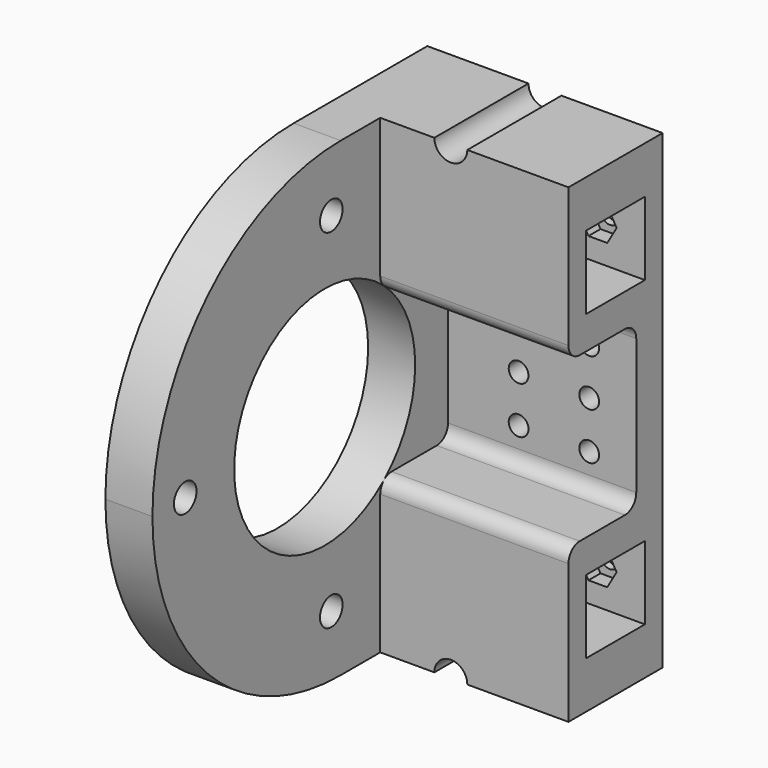
from build123d import *

# Parameters (mm, degrees)
F1_DEPTH     = 100
F2_W         = 15.6
F2_H         = 15.6
F3_DEPTH     = 134.9
F5_DEPTH     = 3.2
F6_R         = 2.025
F7_DEPTH     = 10
F8_R         = 3
F8_R_2       = 24.0417525773
F9_DEPTH     = 15
F10_R        = 49.99999
F11_W        = 18
F11_H        = 34.8
F12_DEPTH    = 100
F13_R        = 3.5
F14_DEPTH    = 50
F15_R        = 2.1
F16_DEPTH    = 25
F17_T1_DEPTH = 47.5
F17_T3_DEPTH = 47.5


# Not quite as in the source:
# - a fillet or chamfer that OpenCascade refuses, or shapes differently, is made with other operations: its cross-section is extruded or revolved along the edge and cut away or added
# - a fillet or chamfer is up to 0.001 mm smaller than in the source, because OpenCascade refuses the exact size


with BuildPart() as f1:
    # F0 (on Top) → F1 (new body)
    with BuildSketch(Plane.XY):
        Polygon((5.1774463622, 16.1983228068), (5.1774463622, 41.1983228068), (-44.8225536378, 41.1983228068), (-44.8225536378, -44.3016771932), (-34.8225536378, -44.3016771932), (-34.8225536378, 16.1983228068), align=None)
    extrude(amount=F1_DEPTH)

    # F2 (on face) → F3 (cut)
    with BuildSketch(Plane.YZ.offset(5.1774463622)):
        with Locations((28.6983228068, 17.8)):
            Rectangle(F2_W, F2_H)
        with Locations((28.6983228068, 82.2)):
            Rectangle(F2_W, F2_H)
    extrude(amount=-F3_DEPTH, mode=Mode.SUBTRACT)

    # F4 (on face) → F5 (cut)
    with BuildSketch(Plane.XZ.offset(-36.4983228068)):
        Polygon((-2.8249217064, 85.66), (-6.8201855692, 85.66), (-8.8178175006, 82.2), (-6.8201855692, 78.74), (-2.8249217064, 78.74), (-0.827289775, 82.2), align=None)
        Polygon((-32.8249217064, 85.66), (-36.8201855692, 85.66), (-38.8178175006, 82.2), (-36.8201855692, 78.74), (-32.8249217064, 78.74), (-30.827289775, 82.2), align=None)
        Polygon((-32.8249217064, 21.26), (-36.8201855692, 21.26), (-38.8178175006, 17.8), (-36.8201855692, 14.34), (-32.8249217064, 14.34), (-30.827289775, 17.8), align=None)
        Polygon((-2.8249217064, 21.26), (-6.8201855692, 21.26), (-8.8178175006, 17.8), (-6.8201855692, 14.34), (-2.8249217064, 14.34), (-0.827289775, 17.8), align=None)
    extrude(amount=-F5_DEPTH, mode=Mode.SUBTRACT)

    # F6 (on face) → F7 (cut)
    with BuildSketch(Plane(origin=(0, 41.1983228068, 0), x_dir=(-1, 0, 0), z_dir=(0, 1, 0))):
        with Locations((34.8225536378, 82.2)):
            Circle(F6_R)
        with Locations((4.8225536378, 17.8)):
            Circle(F6_R)
        with Locations((34.8225536378, 17.8)):
            Circle(F6_R)
        with Locations((4.8225536378, 82.2)):
            Circle(F6_R)
    extrude(amount=-F7_DEPTH, mode=Mode.SUBTRACT)

    # F8 (on face) → F9 (cut)
    with BuildSketch(Plane.YZ.offset(-34.8225536378)):
        with Locations((3.1983228068, 87)):
            Circle(F8_R)
        with Locations((3.1983228068, 13)):
            Circle(F8_R)
        with Locations((-35.6016771932, 50)):
            Circle(F8_R)
        with Locations((1.4400753841, 50)):
            Circle(F8_R_2)
    extrude(amount=-F9_DEPTH, mode=Mode.SUBTRACT)

    # F10 (radius 50 in the source; OpenCascade refuses exactly that, so slightly less here)
    f10_edges = [f1.edges().sort_by_distance(p)[0] for p in [
        (-39.822554, -44.301677, 100),
        (-39.822554, -44.301677, 0),
    ]]
    fillet(f10_edges, radius=F10_R)

    # F11 (on face) → F12 (cut)
    with BuildSketch(Plane.YZ.offset(-34.8225536378)):
        with Locations((25.1983228068, 50)):
            Rectangle(F11_W, F11_H)
    extrude(amount=F12_DEPTH, mode=Mode.SUBTRACT)

    # F13 (on face) → F14 (cut)
    with BuildSketch(Plane(origin=(0, 41.1983228068, 0), x_dir=(-1, 0, 0), z_dir=(0, 1, 0))):
        with Locations((19.8225536378, 0)):
            Circle(F13_R)
        with Locations((19.8225536378, 100)):
            Circle(F13_R)
    extrude(amount=-F14_DEPTH, mode=Mode.SUBTRACT)

    # F15 (on face) → F16 (cut)
    with BuildSketch(Plane(origin=(0, 41.1983228068, 0), x_dir=(-1, 0, 0), z_dir=(0, 1, 0))):
        with Locations((19.8225536378, 50)):
            Circle(F15_R)
        with Locations((19.8225536378, 60)):
            Circle(F15_R)
        with Locations((19.8225536378, 40)):
            Circle(F15_R)
        with Locations((4.8225536378, 50)):
            Circle(F15_R)
        with Locations((4.8225536378, 60)):
            Circle(F15_R)
        with Locations((4.8225536378, 40)):
            Circle(F15_R)
    extrude(amount=-F16_DEPTH, mode=Mode.SUBTRACT)

    # F17: fillet of radius 3 on 4 edges, made by hand

    # F17_s2 → F17_t1 (join)
    with BuildSketch(Plane.YZ.offset(-42.3225536378)):
        with BuildLine():
            ThreePointArc((31.1983228068, 67.4), (33.3196431503, 66.5213203436), (34.1983228068, 64.4))
            Line((34.1983228068, 64.4), (34.1983228068, 67.4))
            Line((34.1983228068, 67.4), (31.1983228068, 67.4))
        make_face()
        with BuildLine():
            ThreePointArc((31.1983228068, 32.6), (33.3196431503, 33.4786796564), (34.1983228068, 35.6))
            Line((34.1983228068, 35.6), (34.1983228068, 32.6))
            Line((34.1983228068, 32.6), (31.1983228068, 32.6))
        make_face()
    extrude(amount=F17_T1_DEPTH)

    # F17_s4 → F17_t3 (cut)
    with BuildSketch(Plane.YZ.offset(-34.8225536378)):
        with BuildLine():
            ThreePointArc((16.1983228068, 70.4), (17.0770024632, 68.2786796564), (19.1983228068, 67.4))
            Line((19.1983228068, 67.4), (16.1983228068, 67.4))
            Line((16.1983228068, 67.4), (16.1983228068, 70.4))
        make_face()
        with BuildLine():
            ThreePointArc((16.1983228068, 29.6), (17.0770024632, 31.7213203436), (19.1983228068, 32.6))
            Line((19.1983228068, 32.6), (16.1983228068, 32.6))
            Line((16.1983228068, 32.6), (16.1983228068, 29.6))
        make_face()
    extrude(amount=F17_T3_DEPTH, mode=Mode.SUBTRACT)


solid = f1.part
